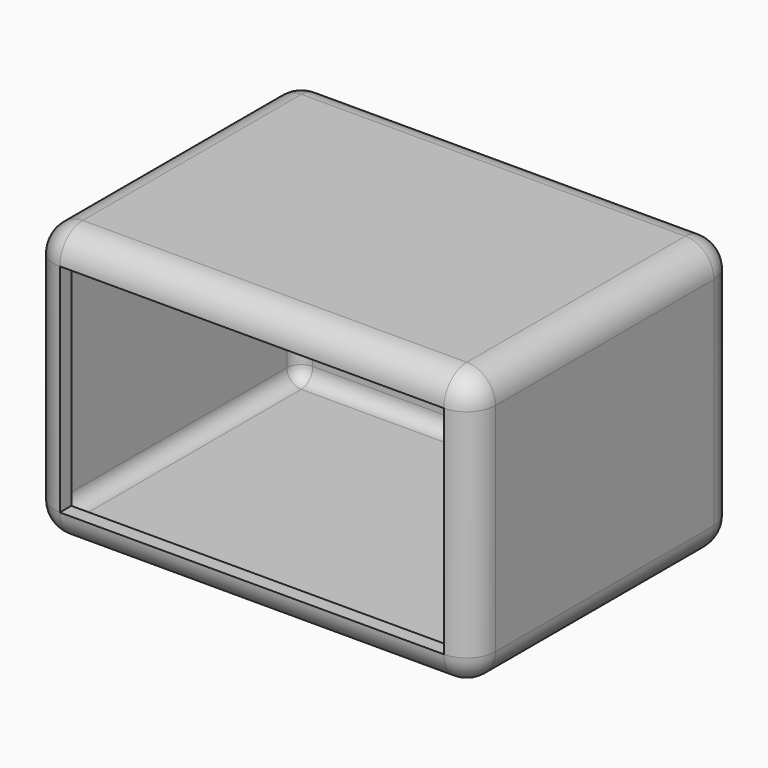
from build123d import *

# Parameters (mm, degrees)
F0_W         = 78.1229734421
F0_H         = 58.4978777915
F1_DEPTH     = 48.514
F2_R         = 5.08
F3_T1_DEPTH  = 67.9629734421
F3_S5_W      = 5.08
F3_S5_H      = 5.08
F3_T6_DEPTH  = 5.08
F3_S11_W     = 5.08
F3_S11_H     = 5.08
F3_T12_DEPTH = 5.08
F4_T         = -2.54


# Not quite as in the source:
# - a fillet or chamfer that OpenCascade refuses, or shapes differently, is made with other operations: its cross-section is extruded or revolved along the edge and cut away or added
# - a shell that OpenCascade refuses in one call is made with other operations: the cavity is built on its own and cut out


with BuildPart() as f1:
    # F0 (on Top) → F1 (new body)
    with BuildSketch(Plane.XY):
        with Locations((-6.4158961177, 8.1142215058)):
            Rectangle(F0_W, F0_H)
    extrude(amount=F1_DEPTH)

    # F2
    f2_edges = [f1.edges().sort_by_distance(p)[0] for p in [
        (-6.415896, -21.134717, 48.514),
        (-45.477383, 8.114222, 48.514),
        (-6.415896, 37.36316, 48.514),
        (32.645591, 8.114222, 48.514),
        (32.645591, -21.134717, 24.257),
        (32.645591, 8.114222, 0),
        (32.645591, 37.36316, 24.257),
        (-45.477383, -21.134717, 24.257),
        (-45.477383, 37.36316, 24.257),
        (-45.477383, 8.114222, 0),
        (-6.415896, 37.36316, 0),
    ]]
    fillet(f2_edges, radius=F2_R)

    # F3: fillet of radius 5.08 on 1 edges, made by hand

    # F3_s2 → F3_t1 (cut)
    with BuildSketch(Plane.YZ.offset(-40.3973828387)):
        with BuildLine():
            ThreePointArc((-16.0547173899, 0), (-19.6468198384, 1.4878975516), (-21.1347173899, 5.08))
            Line((-21.1347173899, 5.08), (-21.1347173899, 0))
            Line((-21.1347173899, 0), (-16.0547173899, 0))
        make_face()
    extrude(amount=F3_T1_DEPTH, mode=Mode.SUBTRACT)


with BuildPart() as f3_tool4:
    # F3_s5 → F3_t6 (new body)
    with BuildSketch(Plane.XY.offset(5.08)):
        with Locations((-42.9373828387, -18.5947173899)):
            Rectangle(F3_S5_W, F3_S5_H)
    extrude(amount=-F3_T6_DEPTH)

    # F3_s7 → F3_t8 (revolve, cut)
    with BuildSketch(Plane(origin=(-40.3973828387, -16.0547173899, 5.08), x_dir=(0.7071067812, 0.7071067812, 0), z_dir=(-0.7071067812, 0.7071067812, 0))):
        with BuildLine():
            ThreePointArc((0, -5.08), (5.08, 0), (0, 5.08))
            Line((0, 5.08), (0, -5.08))
        make_face()
    revolve(axis=Axis((-40.3973828387, -16.0547173899, 5.08), (0, 0, -1)), mode=Mode.SUBTRACT)


with BuildPart() as f1_1:
    add(f1.part)

    # F3_t3: cut F3_tool4
    add(f3_tool4.part, mode=Mode.SUBTRACT)


with BuildPart() as f3_tool10:
    # F3_s11 → F3_t12 (new body)
    with BuildSketch(Plane.XY.offset(5.08)):
        with Locations((30.1055906034, -18.5947173899)):
            Rectangle(F3_S11_W, F3_S11_H)
    extrude(amount=-F3_T12_DEPTH)

    # F3_s13 → F3_t14 (revolve, cut)
    with BuildSketch(Plane(origin=(27.5655906034, -16.0547173899, 5.08), x_dir=(-0.7071067812, 0.7071067812, 0), z_dir=(-0.7071067812, -0.7071067812, 0))):
        with BuildLine():
            ThreePointArc((0, -5.08), (5.08, 0), (0, 5.08))
            Line((0, 5.08), (0, -5.08))
        make_face()
    revolve(axis=Axis((27.5655906034, -16.0547173899, 5.08), (0, 0, -1)), mode=Mode.SUBTRACT)


with BuildPart() as f1_2:
    add(f1_1.part)

    # F3_t9: cut F3_tool10
    add(f3_tool10.part, mode=Mode.SUBTRACT)

    # F4: a shell. OpenCascade refuses it in one call, so the cavity is built on its own and cut out:
    # the body offset inwards by the wall thickness, plus a prism from it out through each open face.
    f4_core = offset(f1_2.part, amount=F4_T, mode=Mode.PRIVATE)
    f4_exits = [f4_core.faces().sort_by_distance(p)[0] for p in [
        (-6.415896, -18.594717, 24.257),
    ]]
    add(f4_core, mode=Mode.SUBTRACT)
    extrude(f4_exits, amount=-F4_T, mode=Mode.SUBTRACT)


solid = f1_2.part
